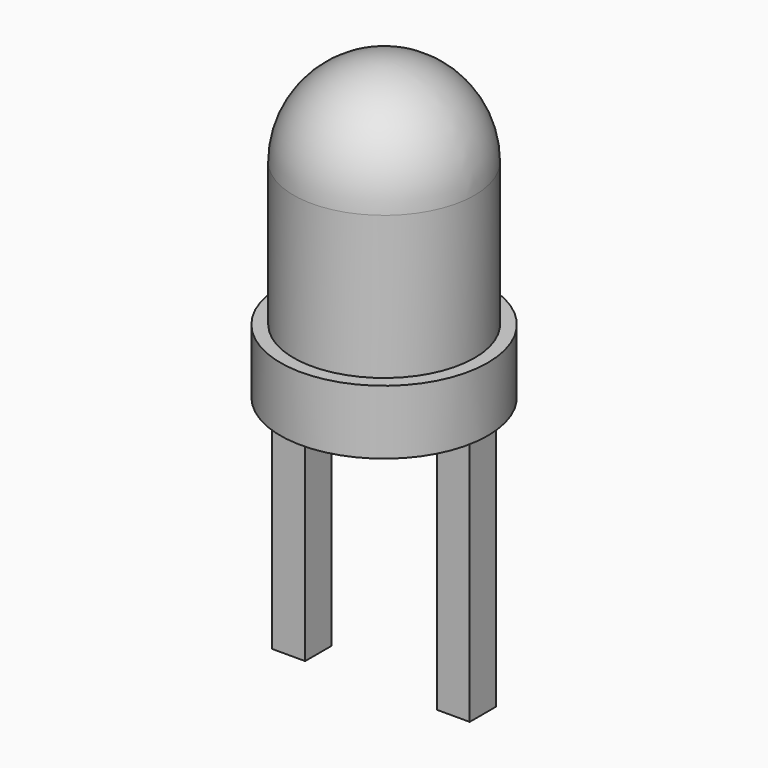
from build123d import *

# Parameters (mm, degrees)
F2_W     = 0.508
F2_H     = 0.508
F3_DEPTH = 3.81


# Not quite as in the source:
# - a pattern or mirror of a feature is missing from the dataset's text; its kind, count and spacing are read off the source's solid


with BuildPart() as f1:
    # F0 (on Front) → F1 (revolve)
    with BuildSketch(Plane.XZ):
        with BuildLine():
            Line((0, 4.5974), (0, 0))
            Line((0, 0), (1.6002, 0))
            Line((1.6002, 0), (1.6002, 0.9906))
            Line((1.6002, 0.9906), (1.397, 0.9906))
            Line((1.397, 0.9906), (1.397, 3.2004))
            ThreePointArc((1.397, 3.2004), (0.9878281733, 4.1882281733), (0, 4.5974))
        make_face()
    revolve(axis=Axis((0, 0, 2.2987), (0, 0, 1)))

    # F2 (on face) → F3 (join)
    with BuildSketch(Plane(origin=(0, 0, 0), x_dir=(1, 0, 0), z_dir=(0, 0, -1))):
        with Locations((1.27, 0)):
            Rectangle(F2_W, F2_H)
    f3 = extrude(amount=F3_DEPTH)

    # F3_copies: F3 across plane
    add(f3.mirror(Plane(origin=(0, 0, 0), x_dir=(0, 0, -1), z_dir=(-1, 0, 0))))


solid = f1.part
